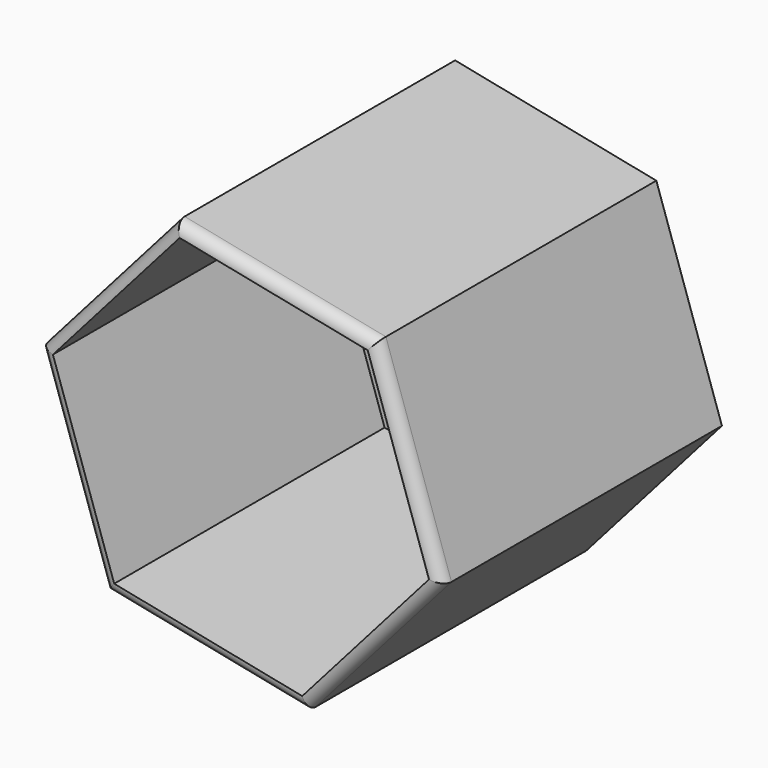
from build123d import *

# Parameters (mm, degrees)
F1_DEPTH = 30
F2_T     = -1
F3_R     = 0.99999


# Not quite as in the source:
# - a fillet or chamfer is up to 0.001 mm smaller than in the source, because OpenCascade refuses the exact size


with BuildPart() as f1:
    # F0 (on Front) → F1 (new body)
    with BuildSketch(Plane.XZ):
        Polygon((-16.0683598468, 10.3036999003), (-4.4305566599, 23.5195108458), (-10.0568830769, 40.2060495226), (-27.3210126808, 43.676777254), (-38.9588158677, 30.4609663085), (-33.3324894507, 13.7744276316), align=None)
    extrude(amount=F1_DEPTH)

    # F2
    f2_openings = [f1.faces().sort_by_distance(p)[0] for p in [
        (-21.694686, -30, 26.990239),
    ]]
    offset(amount=F2_T, openings=f2_openings)

    # F3 (radius 1 in the source; OpenCascade refuses exactly that, so slightly less here)
    f3_edges = [f1.edges().sort_by_distance(p)[0] for p in [
        (-18.688948, -30, 41.941413),
        (-7.24372, -30, 31.86278),
        (-10.249458, -30, 16.911605),
        (-24.700425, -30, 12.039064),
        (-36.145653, -30, 22.117697),
        (-33.139914, -30, 37.068872),
    ]]
    fillet(f3_edges, radius=F3_R)


solid = f1.part
